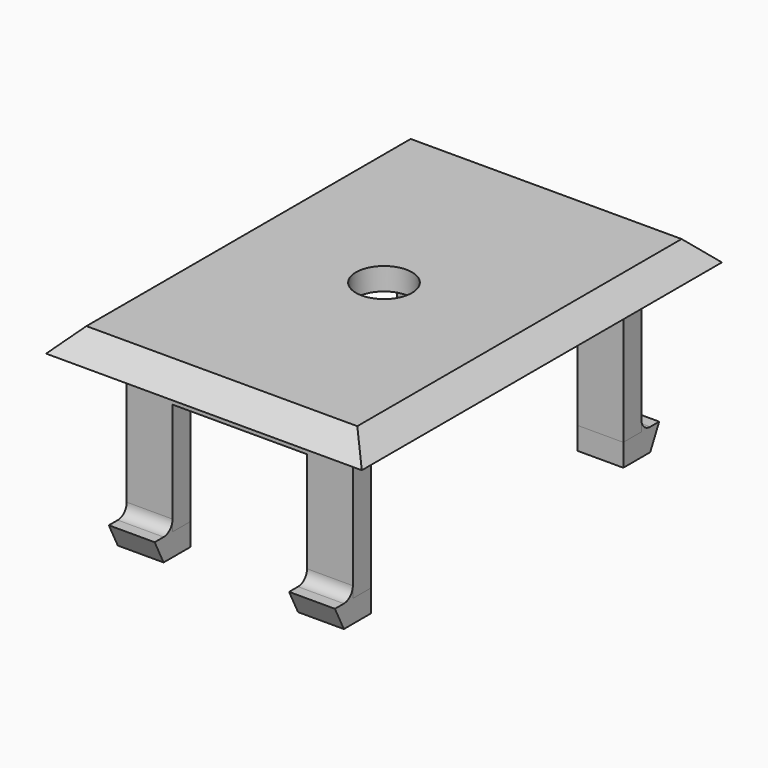
from build123d import *

# Parameters (mm, degrees)
F0_W      = 20.18
F0_H      = 32.18
F0_W_2    = 16.18
F0_H_2    = 28.18
F1_DEPTH  = 13
F2_W      = 28.18
F2_H      = 40.18
F2_W_2    = 20.18
F2_H_2    = 32.18
F2_W_3    = 16.18
F2_H_3    = 28.18
F3_DEPTH  = 2
F4_SIZE   = 1.99999
F6_D      = 5
F8_DEPTH  = 20.18
F9_W      = 28.18
F9_H      = 12
F10_DEPTH = 25
F11_W     = 12
F11_H     = 20
F12_DEPTH = 25


# Not quite as in the source:
# - a fillet or chamfer is up to 0.001 mm smaller than in the source, because OpenCascade refuses the exact size


with BuildPart() as f1:
    # F0 (on Top) → F1 (new body)
    with BuildSketch(Plane.XY):
        Rectangle(F0_W, F0_H)
        Rectangle(F0_W_2, F0_H_2, mode=Mode.SUBTRACT)
    extrude(amount=F1_DEPTH)

    # F2 (on face) → F3 (join)
    with BuildSketch(Plane.XY.offset(13)):
        Rectangle(F2_W, F2_H)
        Rectangle(F2_W_2, F2_H_2, mode=Mode.SUBTRACT)
        Rectangle(F2_W_2, F2_H_2)
        Rectangle(F2_W_3, F2_H_3, mode=Mode.SUBTRACT)
        Rectangle(F2_W_3, F2_H_3)
    extrude(amount=F3_DEPTH)

    # F4 (size 2 in the source; OpenCascade refuses exactly that, so slightly less here)
    f4_edges = [f1.edges().sort_by_distance(p)[0] for p in [
        (0, -20.09, 15),
        (-14.09, 0, 15),
        (0, 20.09, 15),
        (14.09, 0, 15),
    ]]
    chamfer(f4_edges, length=F4_SIZE)

    # F6 (through all)
    with Locations(Plane.XY.offset(15)):
        with Locations((0, 0)):
            Hole(F6_D / 2)


with BuildPart() as f8:
    # F7 (on face) → F8 (new body)
    with BuildSketch(Plane(origin=(-10.09, 0, 0), x_dir=(0, -1, 0), z_dir=(-1, 0, 0))):
        with BuildLine():
            Line((17.09, -2), (18.09, 0))
            Line((18.09, 0), (17.09, 0))
            ThreePointArc((17.09, 0), (16.3828932188, 0.2928932188), (16.09, 1))
            Line((16.09, 1), (16.09, 0))
            Line((16.09, 0), (-16.09, 0))
            Line((-16.09, 0), (-16.09, 1))
            ThreePointArc((-16.09, 1), (-16.3828932188, 0.2928932188), (-17.09, 0))
            Line((-17.09, 0), (-18.09, 0))
            Line((-18.09, 0), (-17.09, -2))
            Line((-17.09, -2), (17.09, -2))
        make_face()
    extrude(amount=-F8_DEPTH)


with BuildPart() as f10_tool:
    # F9 (on face) → F10 (new body)
    with BuildSketch(Plane(origin=(-10.09, 0, 0), x_dir=(0, -1, 0), z_dir=(-1, 0, 0))):
        with Locations((0, 4)):
            Rectangle(F9_W, F9_H)
    extrude(amount=-F10_DEPTH)


with BuildPart() as f1_1:
    add(f1.part)

    # F10: cut by f10_tool
    add(f10_tool.part, mode=Mode.SUBTRACT)


with BuildPart() as f8_1:
    add(f8.part)

    # F10: cut by f10_tool
    add(f10_tool.part, mode=Mode.SUBTRACT)


with BuildPart() as f12_tool:
    # F11 (on Front) → F12 (new body, symmetric)
    with BuildSketch(Plane.XZ):
        Rectangle(F11_W, F11_H)
    extrude(amount=F12_DEPTH, both=True)


with BuildPart() as f1_2:
    add(f1_1.part)

    # F12: cut by f12_tool
    add(f12_tool.part, mode=Mode.SUBTRACT)


with BuildPart() as f8_2:
    add(f8_1.part)

    # F12: cut by f12_tool
    add(f12_tool.part, mode=Mode.SUBTRACT)


solid = Compound([f1_2.part, f8_2.part])
